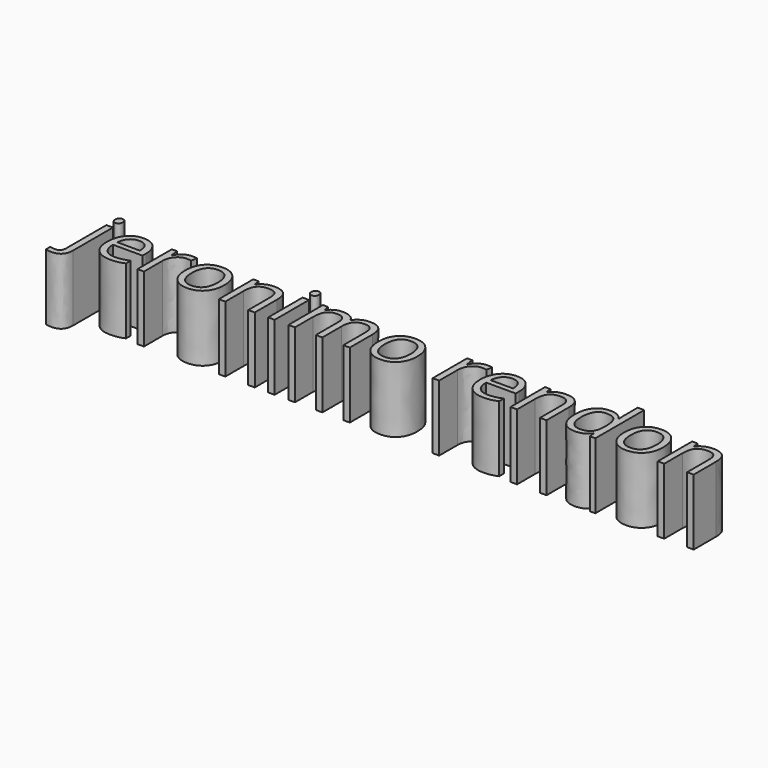
from build123d import *

# Parameters (mm, degrees)
F0_TEXT_SIZE = 16.9177177466
F1_DEPTH     = 13.9


# Not quite as in the source:
# - Text() gives the source's letters only with a copy of the font that has no kerning and outlines rounded to 1/6400 em; it was checked with that copy


with BuildPart() as f1:
    # F0 (on Top) → F1 (new body)
    with BuildSketch(Plane.XY):
        with Locations((-65.8610612154, 39.2333641648)):
            Text('jeronimo rendon', F0_TEXT_SIZE, font='Open Sans', text_align=(TextAlign.LEFT, TextAlign.BOTTOM))
    extrude(amount=F1_DEPTH)


solid = f1.part
